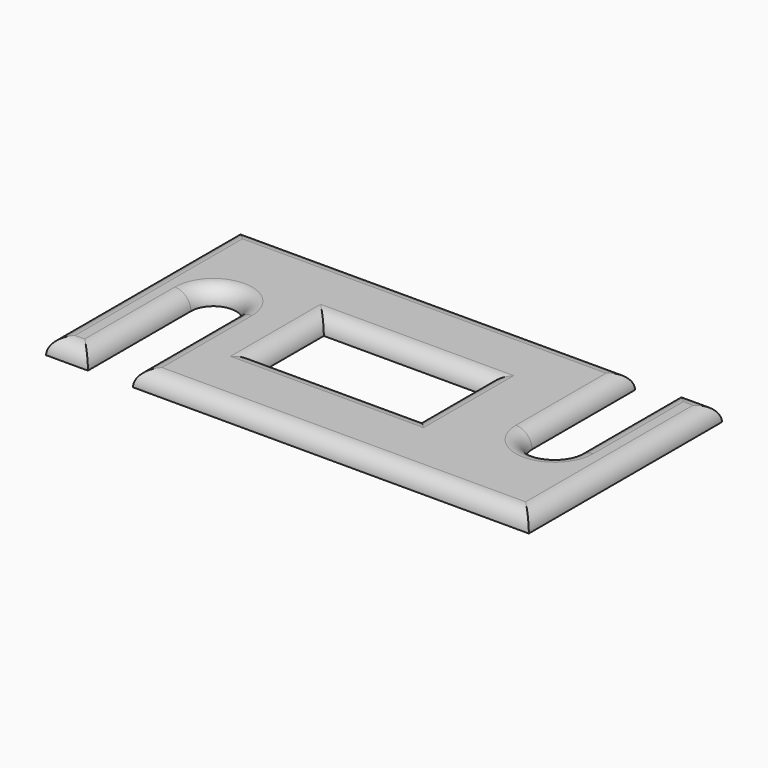
from build123d import *

# Parameters (mm, degrees)
F0_W     = 150
F0_H     = 75
F1_DEPTH = 5
F3_DEPTH = 5.001
F5_DEPTH = 5.001
F6_W     = 50
F6_H     = 25
F7_DEPTH = 5.001
F8_R     = 4.99999


# Not quite as in the source:
# - a fillet or chamfer is up to 0.001 mm smaller than in the source, because OpenCascade refuses the exact size


with BuildPart() as f1:
    # F0 (on Top) → F1 (new body)
    with BuildSketch(Plane.XY):
        with Locations((75, 37.5)):
            Rectangle(F0_W, F0_H)
    extrude(amount=F1_DEPTH)

    # F2 (on face) → F3 (cut, through all)
    with BuildSketch(Plane.XY.offset(5)):
        with BuildLine():
            Line((13, 40), (13, 0))
            Line((13, 0), (27, 0))
            Line((27, 0), (27, 40))
            ThreePointArc((27, 40), (20, 47), (13, 40))
        make_face()
    extrude(amount=-F3_DEPTH, mode=Mode.SUBTRACT)

    # F4 (on face) → F5 (cut, through all)
    with BuildSketch(Plane.XY.offset(5)):
        with BuildLine():
            Line((137, 35), (137, 75))
            Line((137, 75), (123, 75))
            Line((123, 75), (123, 35))
            ThreePointArc((123, 35), (130, 28), (137, 35))
        make_face()
    extrude(amount=-F5_DEPTH, mode=Mode.SUBTRACT)

    # F6 (on face) → F7 (cut, through all)
    with BuildSketch(Plane.XY.offset(5)):
        with Locations((71.2950700867, 37.5)):
            Rectangle(F6_W, F6_H)
    extrude(amount=-F7_DEPTH, mode=Mode.SUBTRACT)

    # F8 (radius 5 in the source; OpenCascade refuses exactly that, so slightly less here)
    f8_edges = [f1.edges().sort_by_distance(p)[0] for p in [
        (88.5, 0, 5),
        (27, 20, 5),
        (150, 37.5, 5),
        (20, 47, 5),
        (143.5, 75, 5),
        (13, 20, 5),
        (137, 55, 5),
        (6.5, 0, 5),
        (130, 28, 5),
        (0, 37.5, 5),
        (123, 55, 5),
        (61.5, 75, 5),
        (71.29507, 50, 5),
        (46.29507, 37.5, 5),
        (71.29507, 25, 5),
        (96.29507, 37.5, 5),
    ]]
    fillet(f8_edges, radius=F8_R)


solid = f1.part
